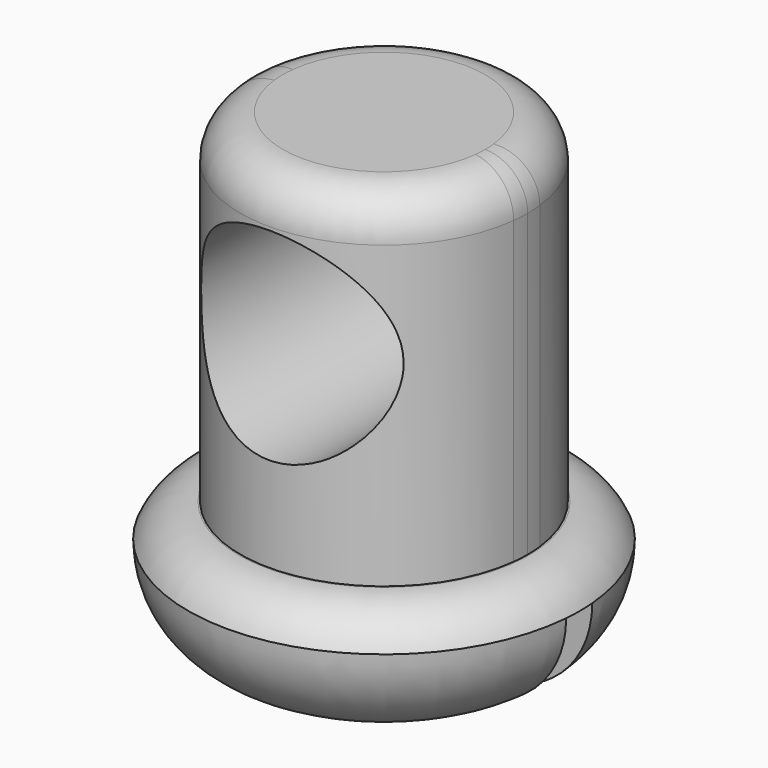
from build123d import *

# Parameters (mm, degrees)
F1_DEPTH = 14.5
F2_DEPTH = 4
F3_DEPTH = 3
F5_R     = 3.1
F6_DEPTH = 10.751
F7_R     = 3
F9_R     = 1.3


# Not quite as in the source:
# - a fillet or chamfer that OpenCascade refuses, or shapes differently, is made with other operations: its cross-section is extruded or revolved along the edge and cut away or added


with BuildPart() as f1:
    # F0 (on Top) → F1 (new body)
    with BuildSketch(Plane.XY):
        with BuildLine():
            Line((-4.3714985989, 0.5), (4.3714985989, 0.5))
            ThreePointArc((4.3714985989, 0.5), (0, 4.4), (-4.3714985989, 0.5))
        make_face()
        with BuildLine():
            ThreePointArc((4.3714985989, -0.5), (4.392868871, -0.2504058355), (4.4, 0))
            ThreePointArc((4.4, 0), (4.392868871, 0.2504058355), (4.3714985989, 0.5))
            Line((4.3714985989, 0.5), (-4.3714985989, 0.5))
            ThreePointArc((-4.3714985989, 0.5), (-4.4, 0), (-4.3714985989, -0.5))
            Line((-4.3714985989, -0.5), (4.3714985989, -0.5))
        make_face()
        with BuildLine():
            ThreePointArc((-4.3714985989, -0.5), (0, -4.4), (4.3714985989, -0.5))
            Line((4.3714985989, -0.5), (-4.3714985989, -0.5))
        make_face()
    extrude(amount=F1_DEPTH)

    # F0 (on Top) → F2 (join)
    with BuildSketch(Plane.XY):
        with BuildLine():
            ThreePointArc((-4.3714985989, -0.5), (-4.4, 0), (-4.3714985989, 0.5))
            Line((-4.3714985989, 0.5), (-5.9791303716, 0.5))
            ThreePointArc((-5.9791303716, 0.5), (-6, 0), (-5.9791303716, -0.5))
            Line((-5.9791303716, -0.5), (-4.3714985989, -0.5))
        make_face()
        with BuildLine():
            Line((5.9791303716, -0.5), (4.3714985989, -0.5))
            ThreePointArc((4.3714985989, -0.5), (0, -4.4), (-4.3714985989, -0.5))
            Line((-4.3714985989, -0.5), (-5.9791303716, -0.5))
            ThreePointArc((-5.9791303716, -0.5), (0, -6), (5.9791303716, -0.5))
        make_face()
        with BuildLine():
            ThreePointArc((4.3714985989, 0.5), (4.392868871, 0.2504058355), (4.4, 0))
            ThreePointArc((4.4, 0), (4.392868871, -0.2504058355), (4.3714985989, -0.5))
            Line((4.3714985989, -0.5), (5.9791303716, -0.5))
            ThreePointArc((5.9791303716, -0.5), (5.9947803225, -0.2502176759), (6, 0))
            ThreePointArc((6, 0), (5.9947803225, 0.2502176759), (5.9791303716, 0.5))
            Line((5.9791303716, 0.5), (4.3714985989, 0.5))
        make_face()
        with BuildLine():
            ThreePointArc((-4.3714985989, 0.5), (0, 4.4), (4.3714985989, 0.5))
            Line((4.3714985989, 0.5), (5.9791303716, 0.5))
            ThreePointArc((5.9791303716, 0.5), (0, 6), (-5.9791303716, 0.5))
            Line((-5.9791303716, 0.5), (-4.3714985989, 0.5))
        make_face()
    extrude(amount=F2_DEPTH)

    # F0 (on Top) → F3 (cut)
    with BuildSketch(Plane.XY):
        with BuildLine():
            ThreePointArc((-4.3714985989, -0.5), (-4.4, 0), (-4.3714985989, 0.5))
            Line((-4.3714985989, 0.5), (-5.9791303716, 0.5))
            ThreePointArc((-5.9791303716, 0.5), (-6, 0), (-5.9791303716, -0.5))
            Line((-5.9791303716, -0.5), (-4.3714985989, -0.5))
        make_face()
        with BuildLine():
            ThreePointArc((4.3714985989, -0.5), (4.392868871, -0.2504058355), (4.4, 0))
            ThreePointArc((4.4, 0), (4.392868871, 0.2504058355), (4.3714985989, 0.5))
            Line((4.3714985989, 0.5), (-4.3714985989, 0.5))
            ThreePointArc((-4.3714985989, 0.5), (-4.4, 0), (-4.3714985989, -0.5))
            Line((-4.3714985989, -0.5), (4.3714985989, -0.5))
        make_face()
        with BuildLine():
            ThreePointArc((4.3714985989, 0.5), (4.392868871, 0.2504058355), (4.4, 0))
            ThreePointArc((4.4, 0), (4.392868871, -0.2504058355), (4.3714985989, -0.5))
            Line((4.3714985989, -0.5), (5.9791303716, -0.5))
            ThreePointArc((5.9791303716, -0.5), (5.9947803225, -0.2502176759), (6, 0))
            ThreePointArc((6, 0), (5.9947803225, 0.2502176759), (5.9791303716, 0.5))
            Line((5.9791303716, 0.5), (4.3714985989, 0.5))
        make_face()
    extrude(amount=F3_DEPTH, mode=Mode.SUBTRACT)

    # F5 (on offset) → F6 (cut, through all)
    with BuildSketch(Plane.XZ.offset(4.75)):
        with Locations((0, 10)):
            Circle(F5_R)
    extrude(amount=-F6_DEPTH, mode=Mode.SUBTRACT)

    # F7
    f7_edges = [f1.edges().sort_by_distance(p)[0] for p in [
        (0, 6, 0),
        (0, -6, 0),
    ]]
    fillet(f7_edges, radius=F7_R)

    # F8: fillet of radius 1.7 on 1 edges, made by hand

    # F8_s1 → F8_t2 (revolve, cut)
    with BuildSketch(Plane(origin=(0, 0, 0), x_dir=(0, 0, 1), z_dir=(0.0833333333, -0.9965217286, 0))):
        with BuildLine():
            ThreePointArc((3, -6), (3.7282856857, -5.3727611072), (4, -4.4508066615))
            Line((4, -4.4508066615), (4.034, -4.4508066615))
            Line((4.034, -4.4508066615), (4.034, -6))
            Line((4.034, -6), (4, -6.034))
            ThreePointArc((4, -6.034), (3.5, -6.034), (3.014, -6.0309838668))
            Line((3.014, -6.0309838668), (3, -6))
        make_face()
    revolve(axis=Axis((0, 0, 4), (0, 0, 1)), mode=Mode.SUBTRACT)

    # F9
    f9_edges = [f1.edges().sort_by_distance(p)[0] for p in [
        (4.371499, 0.5, 14.5),
    ]]
    fillet(f9_edges, radius=F9_R)


solid = f1.part
